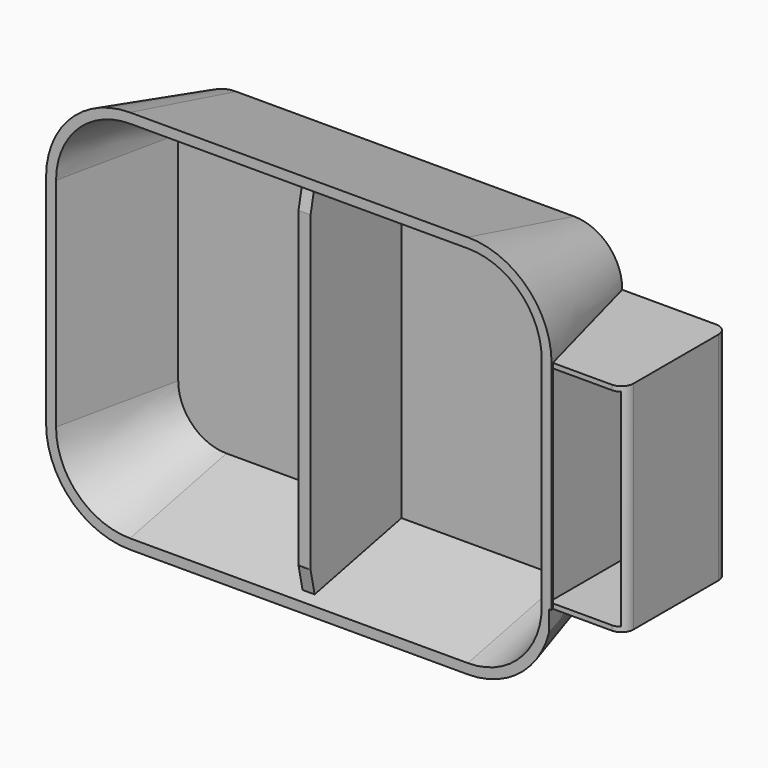
from build123d import *

# Parameters (mm, degrees)
F1_DEPTH     = 55
F1_TAPER     = -15
F4_DEPTH     = 55
F4_TAPER     = -12
F5_W         = 5
F5_H         = 130
F6_DEPTH     = 47
F10_W        = 360.01701653
F10_H        = 225.87454319
F11_DEPTH    = 25
F12_W        = 5
F12_H        = 46
F13_DEPTH    = 10
F14_W        = 5
F14_H        = 46
F15_DEPTH    = 10
F8_W         = 54.0339685977
F8_H         = 90.1
F16_DEPTH    = 32.6
F9_W         = 55.9400806222
F9_H         = 89.7377200425
F17_DEPTH    = 25
F18_W        = 347.7291613817
F18_H        = 217.2330617905
F19_DEPTH    = 25
F20_W        = 34.4053636551
F20_H        = 45.9854951713
F21_DEPTH    = 25
F22_W        = 1.5565819549
F22_H        = 85.7377200425
F22_W_2      = 27.4434180451
F23_DEPTH    = 52
F24_T1_DEPTH = 114.7377200425


# Not quite as in the source:
# - a fillet or chamfer that OpenCascade refuses, or shapes differently, is made with other operations: its cross-section is extruded or revolved along the edge and cut away or added


with BuildPart() as f1:
    # F0 (on Front) → F1 (new body)
    with BuildSketch(Plane.XZ):
        with BuildLine():
            Line((34.0782237053, 85.1892769337), (-105.9217762947, 85.1892769337))
            ThreePointArc((-105.9217762947, 85.1892769337), (-120.0639119184, 79.3314125574), (-125.9217762947, 65.1892769337))
            Line((-125.9217762947, 65.1892769337), (-125.9217762947, -24.8107230663))
            ThreePointArc((-125.9217762947, -24.8107230663), (-120.0639119184, -38.9528586901), (-105.9217762947, -44.8107230663))
            Line((-105.9217762947, -44.8107230663), (34.0782237053, -44.8107230663))
            ThreePointArc((34.0782237053, -44.8107230663), (48.220359329, -38.9528586901), (54.0782237053, -24.8107230663))
            Line((54.0782237053, -24.8107230663), (54.0782237053, 65.1892769337))
            ThreePointArc((54.0782237053, 65.1892769337), (48.220359329, 79.3314125574), (34.0782237053, 85.1892769337))
        make_face()
    extrude(amount=F1_DEPTH, taper=F1_TAPER)

    # F3 (on offset) → F4 (cut)
    with BuildSketch(Plane.XZ.offset(5)):
        with BuildLine():
            Line((34.106137666, 85.2195297501), (-105.893862334, 85.2195297501))
            ThreePointArc((-105.893862334, 85.2195297501), (-120.0359979577, 79.3616653739), (-125.893862334, 65.2195297501))
            Line((-125.893862334, 65.2195297501), (-125.893862334, -24.7804702499))
            ThreePointArc((-125.893862334, -24.7804702499), (-120.0359979577, -38.9226058736), (-105.893862334, -44.7804702499))
            Line((-105.893862334, -44.7804702499), (34.106137666, -44.7804702499))
            ThreePointArc((34.106137666, -44.7804702499), (48.2482732898, -38.9226058736), (54.106137666, -24.7804702499))
            Line((54.106137666, -24.7804702499), (54.106137666, 65.2195297501))
            ThreePointArc((54.106137666, 65.2195297501), (48.2482732898, 79.3616653739), (34.106137666, 85.2195297501))
        make_face()
    extrude(amount=F4_DEPTH, taper=F4_TAPER, mode=Mode.SUBTRACT)

    # F5 (on face) → F6 (join)
    with BuildSketch(Plane.XZ.offset(5)):
        with Locations((-35.893862334, 20.2195297501)):
            Rectangle(F5_W, F5_H)
    extrude(amount=F6_DEPTH)

    # F10 (on Front) → F11 (cut)
    with BuildSketch(Plane.XZ):
        with Locations((5.3876563907, 10.9746605158)):
            Rectangle(F10_W, F10_H)
    extrude(amount=-F11_DEPTH, mode=Mode.SUBTRACT)

    # F12 (on face) → F13 (join)
    with BuildSketch(Plane(origin=(0, 8.8907927165, -41.8278911112), x_dir=(1, 0, 0), z_dir=(0, -0.2079116908, 0.9781476007))):
        with Locations((-35.893862334, -37.2011212889)):
            Rectangle(F12_W, F12_H)
    extrude(amount=F13_DEPTH)

    # F14 (on face) → F15 (join)
    with BuildSketch(Plane(origin=(0, 17.1148163716, 80.5188804202), x_dir=(1, 0, 0), z_dir=(0, -0.2079116908, -0.9781476007))):
        with Locations((-35.893862334, 45.6088745247)):
            Rectangle(F14_W, F14_H)
    extrude(amount=F15_DEPTH)

    # F8 (on offset) → F16 (join)
    with BuildSketch(Plane.YZ.offset(98)):
        with Locations((-27.0169842988, 19.8769969761)):
            Rectangle(F8_W, F8_H)
    extrude(amount=-F16_DEPTH)

    # F9 (on face) → F17 (join)
    with BuildSketch(Plane(origin=(50.4556696128, 13.5195559263, 0), x_dir=(-0.2588190451, 0.9659258263, 0), z_dir=(0.9659258263, 0.2588190451, 0))):
        with Locations((-41.9665145313, 20.0581369549)):
            Rectangle(F9_W, F9_H)
    extrude(amount=F17_DEPTH)

    # F18 (on Front) → F19 (cut)
    with BuildSketch(Plane.XZ):
        with Locations((0.111065805, 20.1892703772)):
            Rectangle(F18_W, F18_H)
    extrude(amount=-F19_DEPTH, mode=Mode.SUBTRACT)

    # F20 (on face) → F21 (cut)
    with BuildSketch(Plane(origin=(0, 0, -24.8107230663), x_dir=(1, 0, 0), z_dir=(0, 0, -1))):
        Polygon((68.0166854944, 55.7510983837), (65.4, 45.9854951713), (99.8053636551, 45.9854951713), (100.283839941, 55.7510983837), align=None)
        with Locations((82.6026818275, 22.9927475857)):
            Rectangle(F20_W, F20_H)
    extrude(amount=F21_DEPTH, mode=Mode.SUBTRACT)

    # F22 (on face) → F23 (cut)
    with BuildSketch(Plane.XZ.offset(54.0339685977)):
        with Locations((67.7782909774, 20.0581369549)):
            Rectangle(F22_W, F22_H)
        with Locations((82.2782909774, 20.0581369549)):
            Rectangle(F22_W_2, F22_H)
    extrude(amount=-F23_DEPTH, mode=Mode.SUBTRACT)

    # F24: fillet of radius 5 on 2 edges, made by hand

    # F24_s2 → F24_t1 (cut)
    with BuildSketch(Plane.XY.offset(-37.3107230663)):
        with BuildLine():
            ThreePointArc((98, -49.0339685977), (96.5355339059, -52.5695025036), (93, -54.0339685977))
            Line((93, -54.0339685977), (98, -54.0339685977))
            Line((98, -54.0339685977), (98, -49.0339685977))
        make_face()
        with BuildLine():
            ThreePointArc((93, 0), (96.5355339059, -1.4644660941), (98, -5))
            Line((98, -5), (98, 0))
            Line((98, 0), (93, 0))
        make_face()
    extrude(amount=F24_T1_DEPTH, mode=Mode.SUBTRACT)


solid = f1.part
